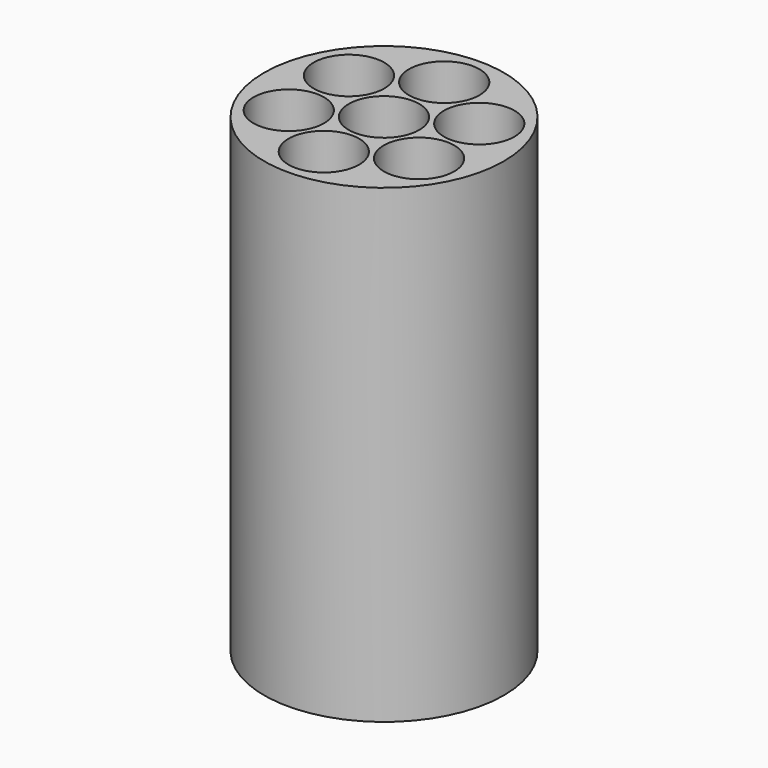
from build123d import *

# Parameters (mm, degrees)
F2_R         = 1.275
F3_DEPTH     = 5
F1_R         = 0.375
F4_DEPTH     = 5.001
F9_TEXT_SIZE = 4.0725106373
F10_DEPTH    = 0.2


# Not quite as in the source:
# - Text() gives the source's letters only with a copy of the font that has no kerning and outlines rounded to 1/6400 em; it was checked with that copy


with BuildPart() as f3:
    # F2 (on Top) → F3 (new body)
    with BuildSketch(Plane.XY):
        Circle(F2_R)
    extrude(amount=F3_DEPTH)

    # F1 (on Top) → F4 (cut, through all)
    with BuildSketch(Plane.XY):
        Circle(F1_R)
        with Locations((0, 0.8)):
            Circle(F1_R)
        with Locations((0.692820323, 0.4)):
            Circle(F1_R)
        with Locations((0.692820323, -0.4)):
            Circle(F1_R)
        with Locations((0, -0.8)):
            Circle(F1_R)
        with Locations((-0.692820323, -0.4)):
            Circle(F1_R)
        with Locations((-0.692820323, 0.4)):
            Circle(F1_R)
    extrude(amount=F4_DEPTH, mode=Mode.SUBTRACT)

    # F9 (on face) → F10 (join)
    with BuildSketch(Plane(origin=(0, 1.175, 0), x_dir=(-1, 0, 0), z_dir=(0, 1, 0))):
        with Locations((-0.5306211824, 0.9909162764)):
            Text('I', F9_TEXT_SIZE, font='Open Sans', text_align=(TextAlign.LEFT, TextAlign.BOTTOM))
    extrude(amount=F10_DEPTH)


solid = f3.part
